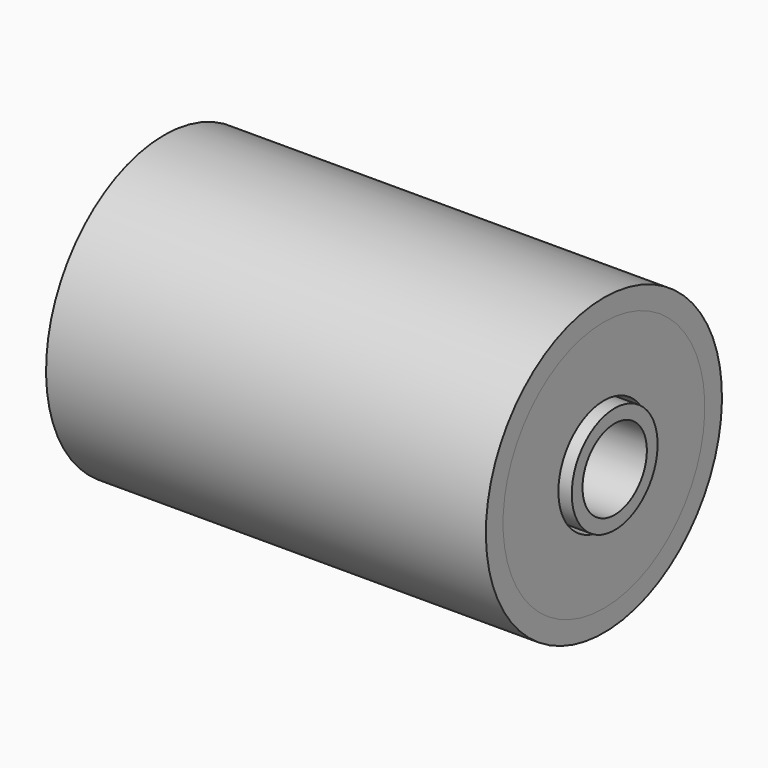
from build123d import *

# Parameters (mm, degrees)
F3_R     = 4.7625
F4_DEPTH = 25.4


# Not quite as in the source:
# - a feature names something its author has since deleted; it is built from what else it names


with BuildPart() as f1:
    # F0 (on Front) → F1 (revolve)
    with BuildSketch(Plane.XZ):
        Polygon((-12.7, 0), (0, 0), (9.525, 0), (14.605, 0), (14.605, 6.35), (9.525, 6.35), (0, 6.35), (0, 11.43), (-12.7, 11.43), (-12.7, 7.493), (-21.6916, 7.493), (-21.6916, 5.7102125138), (-20.9189541638, 5.7102125138), (-20.9189541638, 3.9878), (-21.6916, 3.9878), (-28.702, 3.9878), (-28.702, 0), (-27.686, 0), (-26.6954, 0), (-21.6916, 0), align=None)
    revolve(axis=Axis((-24.1935, 0, 0), (-1, 0, 0)))

    # F3 (on face) → F4 (cut)
    with BuildSketch(Plane.YZ.offset(14.605)):
        Circle(F3_R)
    extrude(amount=-F4_DEPTH, mode=Mode.SUBTRACT)


with BuildPart() as f2:
    # F0 (on Front) → F2 (revolve)
    with BuildSketch(Plane.XZ):
        Polygon((0, 6.35), (9.525, 6.35), (9.525, 13.2726598531), (9.525, 14.2875), (0, 14.2875), (0, 12.7320755273), (0, 11.43), align=None)
    revolve(axis=Axis((0, 0, 0), (-1, 0, 0)))


with BuildPart() as f2b:
    # F0 (on Front) → F2, piece 2 (revolve)
    with BuildSketch(Plane.XZ):
        Polygon((-12.7, 7.493), (-12.7, 11.43), (-12.7, 12.7320755273), (-12.7, 13.9954), (-21.6916, 13.9954), (-21.6916, 10.9982), (-21.6916, 7.493), align=None)
    revolve(axis=Axis((0, 0, 0), (-1, 0, 0)))


with BuildPart() as f5:
    # F0 (on Front) → F5 (revolve)
    with BuildSketch(Plane.XZ):
        Polygon((0, 14.2875), (9.525, 14.2875), (9.525, 14.9225), (9.525, 16.1469075829), (10.7906318894, 16.1469075829), (10.7906318894, 14.9225), (13.3306318894, 14.9225), (13.3306318894, 17.4625), (-37.4693681106, 17.4625), (-38.7236513197, 17.4625), (-38.7236513197, 0), (-37.4693681106, 0), (-32.7810309827, 0), (-32.7628890359, 3.9878), (-30.2228890359, 3.9878), (-30.2228890359, 10.9982), (-28.702, 10.9982), (-27.686, 10.9982), (-21.6916, 10.9982), (-21.6916, 13.9954), (-12.7, 13.9954), (-12.7, 12.7320755273), (0, 12.7320755273), align=None)
    revolve(axis=Axis((-12.7, 0, 0), (-1, 0, 0)))


with BuildPart() as f6:
    # F0 (on Front) → F6 (revolve)
    with BuildSketch(Plane.XZ):
        Polygon((9.525, 14.2875), (9.525, 13.2726598531), (10.285962373, 13.2726598531), (10.285962373, 7.4942293577), (10.285962373, 6.7371539772), (13.3306318894, 6.7371539772), (13.3306318894, 7.4942293577), (13.3306318894, 14.9225), (10.7906318894, 14.9225), (9.525, 14.9225), align=None)
    revolve(axis=Axis((14.605, 0, 0), (-1, 0, 0)))


with BuildPart() as f7:
    # F0 (on Front) → F7 (revolve)
    with BuildSketch(Plane.XZ):
        Polygon((-28.702, 10.9982), (-28.702, 3.9878), (-21.6916, 3.9878), (-21.6916, 5.7102125138), (-21.6916, 7.493), (-21.6916, 10.9982), (-27.686, 10.9982), align=None)
    revolve(axis=Axis((13.3306318894, 0, 0), (-1, 0, 0)))


solid = Compound([f1.part, f2.part, f2b.part, f5.part, f6.part, f7.part])
